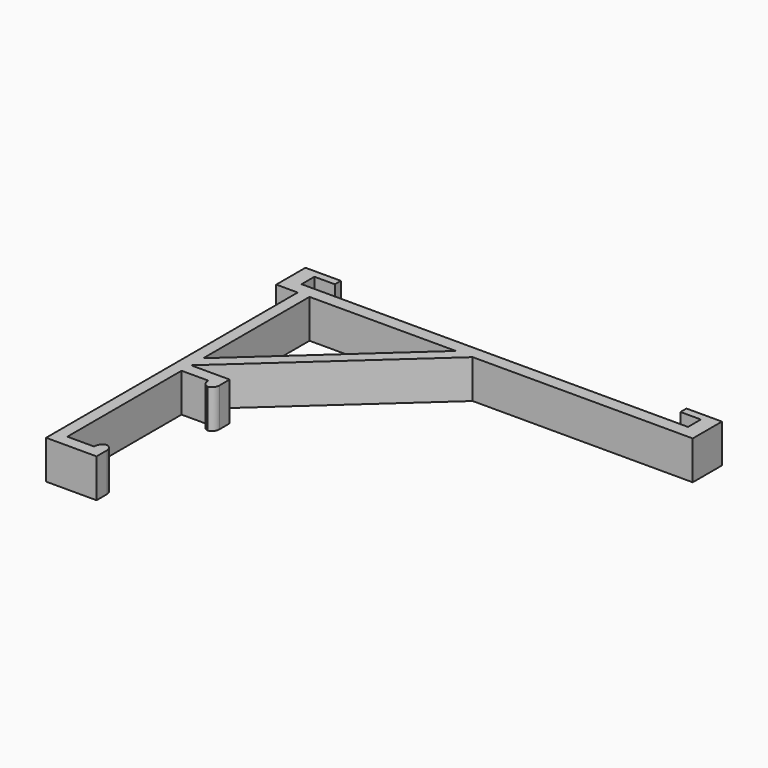
from build123d import *

# Parameters (mm, degrees)
F1_DEPTH    = 9.144
F2_T1_DEPTH = 18.034


# Not quite as in the source:
# - a fillet or chamfer that OpenCascade refuses, or shapes differently, is made with other operations: its cross-section is extruded or revolved along the edge and cut away or added


with BuildPart() as f1:
    # F0 (on Top) → F1 (new body)
    with BuildSketch(Plane.XY):
        Polygon((-45.8869487338, 19.8141042413), (-45.8869487338, 21.5921042413), (-54.2689487338, 21.5921042413), (-54.2689487338, 12.9561042413), (-49.1889487338, 12.9561042413), (-49.1889487338, -61.4658957587), (-37.2509487338, -61.4658957587), (-37.2509487338, -56.6398957587), (-40.0449487338, -56.6398957587), (-40.0449487338, -58.6718957587), (-46.3949487338, -58.6718957587), (-46.3949487338, -37.378154695), (-46.3949487338, -27.9378957587), (-46.3949487338, -24.8898957587), (-40.0449487338, -24.8898957587), (-40.0449487338, -26.9218957587), (-37.2509487338, -26.9218957587), (-37.2509487338, -22.0958957587), (-46.3949487338, -22.0958957587), (-7.7869487338, 12.9561042413), (44.2830512662, 12.9561042413), (44.2830512662, 21.5921042413), (35.9010512662, 21.5921042413), (35.9010512662, 19.8141042413), (40.7270512662, 19.8141042413), (40.7270512662, 16.0041042413), (-50.7129487338, 16.0041042413), (-50.7129487338, 19.8141042413), align=None)
        Polygon((-11.7646907362, 12.9561042413), (-46.3949487338, -18.4845247302), (-46.3949487338, 12.9561042413), align=None, mode=Mode.SUBTRACT)
    extrude(amount=F1_DEPTH)

    # F2: fillet of radius 1.778 on 4 edges, made by hand

    # F2_s2 → F2_t1 (cut)
    with BuildSketch(Plane.XY.offset(-4.445)):
        with BuildLine():
            ThreePointArc((-38.2669487338, -26.9218957587), (-39.5241845908, -26.4011316156), (-40.0449487338, -25.1438957587))
            Line((-40.0449487338, -25.1438957587), (-40.0449487338, -26.9218957587))
            Line((-40.0449487338, -26.9218957587), (-38.2669487338, -26.9218957587))
        make_face()
        with BuildLine():
            ThreePointArc((-37.2509487338, -25.1438957587), (-37.7717128769, -26.4011316156), (-39.0289487338, -26.9218957587))
            Line((-39.0289487338, -26.9218957587), (-37.2509487338, -26.9218957587))
            Line((-37.2509487338, -26.9218957587), (-37.2509487338, -25.1438957587))
        make_face()
        with BuildLine():
            ThreePointArc((-39.0289487338, -56.6398957587), (-37.7717128769, -57.1606599017), (-37.2509487338, -58.4178957587))
            Line((-37.2509487338, -58.4178957587), (-37.2509487338, -56.6398957587))
            Line((-37.2509487338, -56.6398957587), (-39.0289487338, -56.6398957587))
        make_face()
        with BuildLine():
            ThreePointArc((-40.0449487338, -58.4178957587), (-39.5241845908, -57.1606599017), (-38.2669487338, -56.6398957587))
            Line((-38.2669487338, -56.6398957587), (-40.0449487338, -56.6398957587))
            Line((-40.0449487338, -56.6398957587), (-40.0449487338, -58.4178957587))
        make_face()
    extrude(amount=F2_T1_DEPTH, mode=Mode.SUBTRACT)


solid = f1.part
